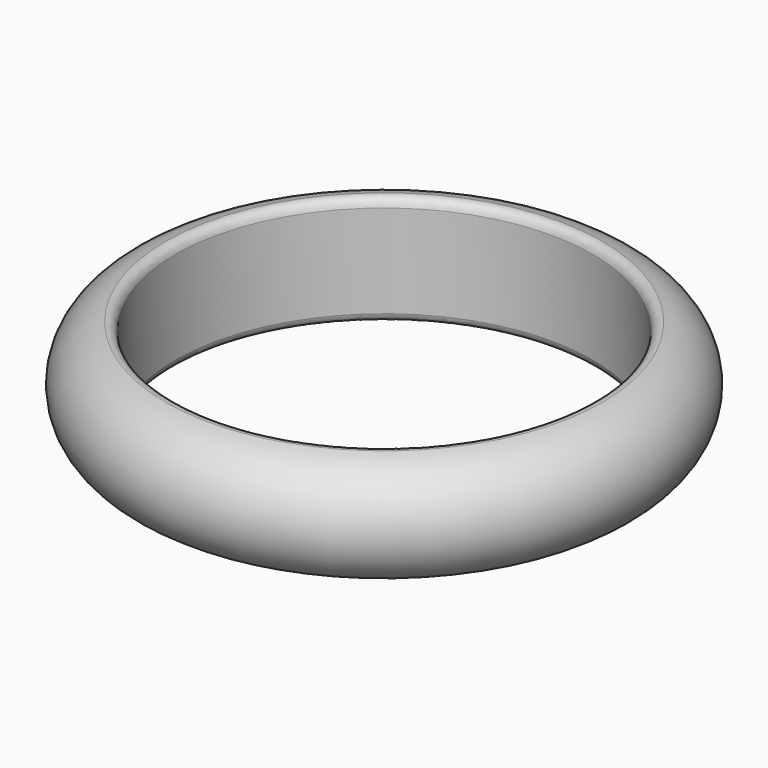
from build123d import *

# Parameters (mm, degrees)
F3_R = 0.3


with BuildPart() as f2:
    # F2: sweep along a path in F0
    with BuildLine(Plane.XY) as f2_path:
        CenterArc((0, 0), 7.5, 0, 360)
    # F1 (on Front) → F2 (sweep)
    with BuildSketch(Plane.XZ):
        with BuildLine():
            Line((7.5, 4), (7.5, 0))
            ThreePointArc((7.5, 0), (9.5, 2), (7.5, 4))
        make_face()
    sweep(path=f2_path.line)

    # F3
    f3_edges = [f2.edges().sort_by_distance(p)[0] for p in [
        (-7.5, 0, 4),
        (-7.5, 0, 0),
    ]]
    fillet(f3_edges, radius=F3_R)


solid = f2.part
